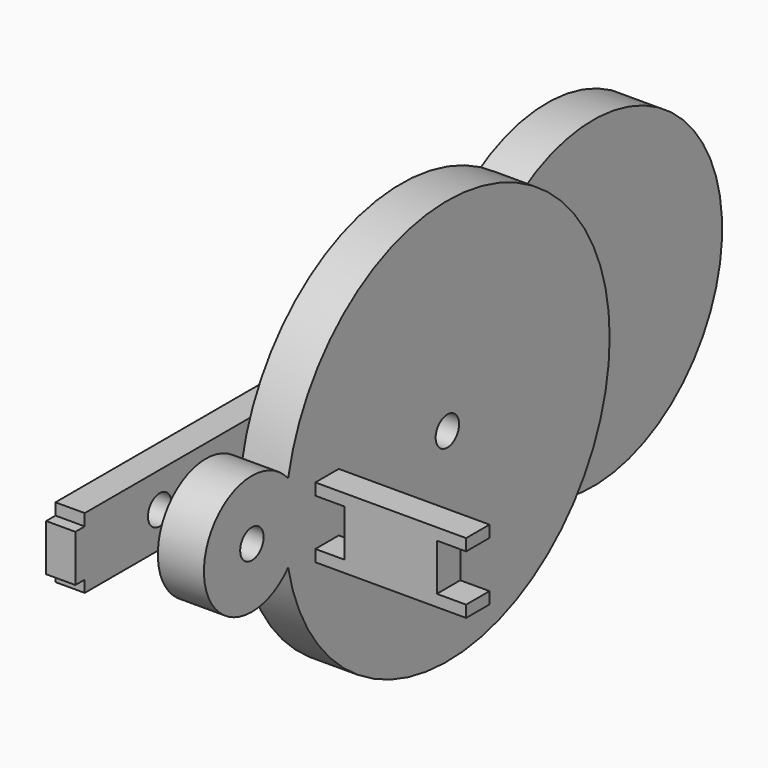
from build123d import *

# Parameters (mm, degrees)
F0_R     = 4.5
F0_R_2   = 1.5875
F1_DEPTH = 5
F2_R     = 1.5875
F3_DEPTH = 5
F4_R     = 1.5875
F4_W     = 1.27
F4_H     = 2.54
F5_DEPTH = 3.175
F7_DEPTH = 3.175


with BuildPart() as f1:
    # F0 (on Right) → F1 (new body)
    with BuildSketch(Plane.YZ):
        with BuildLine():
            ThreePointArc((4.9150943396, 4.2534512613), (6.0908994905, 2.2695689891), (6.5, 0))
            ThreePointArc((6.5, 0), (6.0908994905, -2.2695689891), (4.9150943396, -4.2534512613))
            ThreePointArc((4.9150943396, -4.2534512613), (28.6368288972, -21.8959805047), (48.5, 0))
            ThreePointArc((48.5, 0), (28.6368288972, 21.8959805047), (4.9150943396, 4.2534512613))
        make_face()
        with BuildLine():
            ThreePointArc((46.5, 0), (26.5, -20), (6.5, 0))
            ThreePointArc((6.5, 0), (26.5, 20), (46.5, 0))
        make_face(mode=Mode.SUBTRACT)
        with BuildLine():
            ThreePointArc((46.5, 0), (26.5, 20), (6.5, 0))
            ThreePointArc((6.5, 0), (26.5, -20), (46.5, 0))
        make_face()
        with BuildLine():
            ThreePointArc((28.0875, 0), (26.5, -1.5875), (24.9125, 0))
            ThreePointArc((24.9125, 0), (26.5, 1.5875), (28.0875, 0))
        make_face(mode=Mode.SUBTRACT)
        with BuildLine():
            ThreePointArc((4.5, 0), (4.6040194953, 2.1368288972), (4.9150943396, 4.2534512613))
            ThreePointArc((4.9150943396, 4.2534512613), (-6.5, 0), (4.9150943396, -4.2534512613))
            ThreePointArc((4.9150943396, -4.2534512613), (4.6040194953, -2.1368288972), (4.5, 0))
        make_face()
        Circle(F0_R, mode=Mode.SUBTRACT)
        Circle(F0_R)
        Circle(F0_R_2, mode=Mode.SUBTRACT)
        with BuildLine():
            Line((4.5, 0), (6.5, 0))
            ThreePointArc((6.5, 0), (6.0908994905, 2.2695689891), (4.9150943396, 4.2534512613))
            ThreePointArc((4.9150943396, 4.2534512613), (4.6040194953, 2.1368288972), (4.5, 0))
        make_face()
        with BuildLine():
            ThreePointArc((4.9150943396, -4.2534512613), (6.0908994905, -2.2695689891), (6.5, 0))
            Line((6.5, 0), (4.5, 0))
            ThreePointArc((4.5, 0), (4.6040194953, -2.1368288972), (4.9150943396, -4.2534512613))
        make_face()
    extrude(amount=F1_DEPTH)

    # F2 (on face) → F3 (join)
    with BuildSketch(Plane(origin=(0, 0, 0), x_dir=(0, -1, 0), z_dir=(-1, 0, 0))):
        with BuildLine():
            ThreePointArc((-44.1875, -13.0825205427), (-47.3940781084, -6.887488657), (-48.5, 0))
            ThreePointArc((-48.5, 0), (-47.3940781084, 6.887488657), (-44.1875, 13.0825205427))
            ThreePointArc((-44.1875, 13.0825205427), (-68, 0), (-44.1875, -13.0825205427))
        make_face()
        with Locations((-52.5, 0)):
            Circle(F2_R, mode=Mode.SUBTRACT)
        with BuildLine():
            ThreePointArc((-35.7307692308, 5.004288102), (-35.1836560085, 2.5286816267), (-35, 0))
            ThreePointArc((-35, 0), (-35.1836560085, -2.5286816267), (-35.7307692308, -5.004288102))
            ThreePointArc((-35.7307692308, -5.004288102), (-23.9186318476, -10.1777472194), (-16, 0))
            ThreePointArc((-16, 0), (-23.9186318476, 10.1777472194), (-35.7307692308, 5.004288102))
        make_face()
        with BuildLine():
            ThreePointArc((-35, 0), (-26.5, 8.5), (-18, 0))
            ThreePointArc((-18, 0), (-26.5, -8.5), (-35, 0))
        make_face(mode=Mode.SUBTRACT)
        with BuildLine():
            ThreePointArc((-35, 0), (-26.5, -8.5), (-18, 0))
            ThreePointArc((-18, 0), (-26.5, 8.5), (-35, 0))
        make_face()
        with BuildLine():
            ThreePointArc((-24.9125, 0), (-26.5, -1.5875), (-28.0875, 0))
            ThreePointArc((-28.0875, 0), (-26.5, 1.5875), (-24.9125, 0))
        make_face(mode=Mode.SUBTRACT)
        with BuildLine():
            ThreePointArc((-44.1875, -13.0825205427), (-68, 0), (-44.1875, 13.0825205427))
            ThreePointArc((-44.1875, 13.0825205427), (-43.5707428158, 13.8776705436), (-42.9182692308, 14.643784875))
            ThreePointArc((-42.9182692308, 14.643784875), (-70, 0), (-42.9182692308, -14.643784875))
            ThreePointArc((-42.9182692308, -14.643784875), (-43.5707428158, -13.8776705436), (-44.1875, -13.0825205427))
        make_face()
        with BuildLine():
            ThreePointArc((-44.1875, -13.0825205427), (-38.9151969098, -7.4634526193), (-37, 0))
            Line((-37, 0), (-48.5, 0))
            ThreePointArc((-48.5, 0), (-47.3940781084, -6.887488657), (-44.1875, -13.0825205427))
        make_face()
        with BuildLine():
            Line((-48.5, 0), (-37, 0))
            ThreePointArc((-37, 0), (-38.9151969098, 7.4634526193), (-44.1875, 13.0825205427))
            ThreePointArc((-44.1875, 13.0825205427), (-47.3940781084, 6.887488657), (-48.5, 0))
        make_face()
        with BuildLine():
            ThreePointArc((-44.1875, 13.0825205427), (-38.9151969098, 7.4634526193), (-37, 0))
            ThreePointArc((-37, 0), (-36.6777472194, 2.5813681524), (-35.7307692308, 5.004288102))
            ThreePointArc((-35.7307692308, 5.004288102), (-38.4706283815, 10.4607233015), (-42.9182692308, 14.643784875))
            ThreePointArc((-42.9182692308, 14.643784875), (-43.5707428158, 13.8776705436), (-44.1875, 13.0825205427))
        make_face()
        with BuildLine():
            ThreePointArc((-35.7307692308, -5.004288102), (-36.6777472194, -2.5813681524), (-37, 0))
            ThreePointArc((-37, 0), (-38.9151969098, -7.4634526193), (-44.1875, -13.0825205427))
            ThreePointArc((-44.1875, -13.0825205427), (-43.5707428158, -13.8776705436), (-42.9182692308, -14.643784875))
            ThreePointArc((-42.9182692308, -14.643784875), (-38.4706283815, -10.4607233015), (-35.7307692308, -5.004288102))
        make_face()
        with BuildLine():
            ThreePointArc((-35.7307692308, -5.004288102), (-35.1836560085, -2.5286816267), (-35, 0))
            Line((-35, 0), (-37, 0))
            ThreePointArc((-37, 0), (-36.6777472194, -2.5813681524), (-35.7307692308, -5.004288102))
        make_face()
        with BuildLine():
            Line((-37, 0), (-35, 0))
            ThreePointArc((-35, 0), (-35.1836560085, 2.5286816267), (-35.7307692308, 5.004288102))
            ThreePointArc((-35.7307692308, 5.004288102), (-36.6777472194, 2.5813681524), (-37, 0))
        make_face()
    extrude(amount=F3_DEPTH)


with BuildPart() as f5:
    # F4 (on face) → F5 (new body)
    with BuildSketch(Plane(origin=(-5, 0, 0), x_dir=(0, -1, 0), z_dir=(-1, 0, 0))):
        with BuildLine():
            ThreePointArc((-69.5802195536, 3.81), (-69.8947383163, 1.9165278255), (-70, 0))
            ThreePointArc((-70, 0), (-69.8947383163, -1.9165278255), (-69.5802195536, -3.81))
            Line((-69.5802195536, -3.81), (-16.7156298108, -3.81))
            ThreePointArc((-16.7156298108, -3.81), (-16, 0), (-16.7156298108, 3.81))
            Line((-16.7156298108, 3.81), (-69.5802195536, 3.81))
        make_face()
        with BuildLine():
            ThreePointArc((-54.0875, 0), (-52.5, 1.5875), (-50.9125, 0))
            ThreePointArc((-50.9125, 0), (-52.5, -1.5875), (-54.0875, 0))
        make_face(mode=Mode.SUBTRACT)
        with Locations((-26.5, 0)):
            Circle(F4_R, mode=Mode.SUBTRACT)
        with BuildLine():
            Line((-72.54, 0), (-70, 0))
            ThreePointArc((-70, 0), (-69.8947383163, 1.9165278255), (-69.5802195536, 3.81))
            Line((-69.5802195536, 3.81), (-72.54, 3.81))
            Line((-72.54, 3.81), (-72.54, 2.54))
            Line((-72.54, 2.54), (-72.54, 0))
        make_face()
        with BuildLine():
            ThreePointArc((-69.5802195536, -3.81), (-69.8947383163, -1.9165278255), (-70, 0))
            Line((-70, 0), (-72.54, 0))
            Line((-72.54, 0), (-72.54, -2.54))
            Line((-72.54, -2.54), (-72.54, -3.81))
            Line((-72.54, -3.81), (-69.5802195536, -3.81))
        make_face()
        with Locations((-73.175, -1.27)):
            Rectangle(F4_W, F4_H)
        with Locations((-73.175, 1.27)):
            Rectangle(F4_W, F4_H)
        with BuildLine():
            Line((10.16, 3.81), (-16.7156298108, 3.81))
            ThreePointArc((-16.7156298108, 3.81), (-16, 0), (-16.7156298108, -3.81))
            Line((-16.7156298108, -3.81), (0, -3.81))
            Line((0, -3.81), (10.16, -3.81))
            Line((10.16, -3.81), (10.16, -2.54))
            Line((10.16, -2.54), (10.16, 0))
            Line((10.16, 0), (10.16, 2.54))
            Line((10.16, 2.54), (10.16, 3.81))
        make_face()
        Circle(F4_R, mode=Mode.SUBTRACT)
        with Locations((10.795, 1.27)):
            Rectangle(F4_W, F4_H)
        with Locations((10.795, -1.27)):
            Rectangle(F4_W, F4_H)
    extrude(amount=F5_DEPTH)


with BuildPart() as f7:
    # F6 (on Front) → F7 (new body)
    with BuildSketch(Plane.XZ):
        Polygon((30.7720199436, 8.9457957841), (30.7720199436, 10.2157957841), (22.5970199436, 10.2157957841), (22.5970199436, 2.5957957841), (30.7720199436, 2.5957957841), (30.7720199436, 3.8657957841), (27.5970199436, 3.8657957841), (27.5970199436, 8.9457957841), align=None)
        Polygon((22.5970199436, 2.5957957841), (22.5970199436, 10.2157957841), (14.4220199436, 10.2157957841), (14.4220199436, 8.9457957841), (17.5970199436, 8.9457957841), (17.5970199436, 3.8657957841), (14.4220199436, 3.8657957841), (14.4220199436, 2.5957957841), align=None)
    extrude(amount=F7_DEPTH)


solid = Compound([f1.part, f5.part, f7.part])
